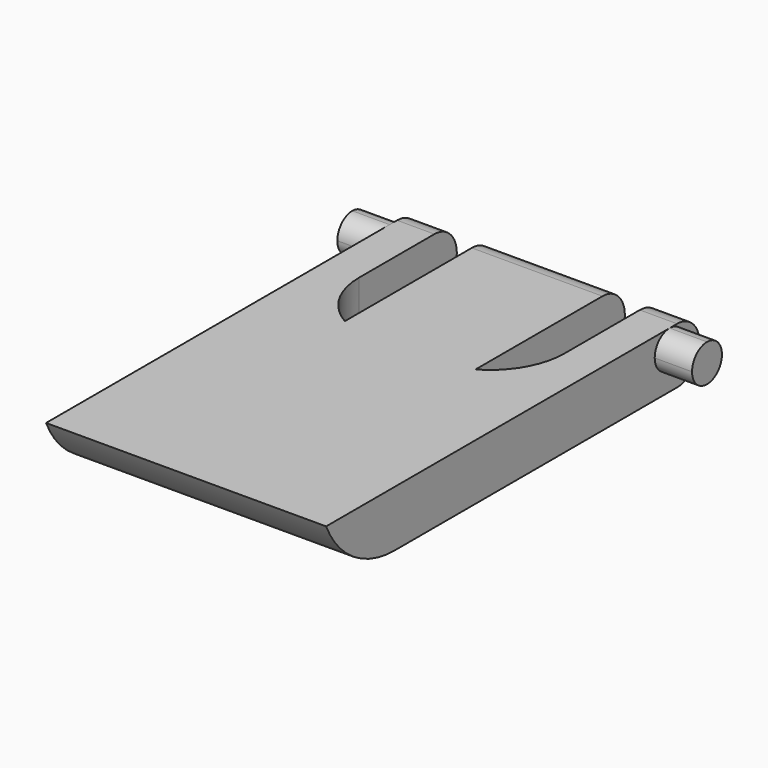
from build123d import *

# Parameters (mm, degrees)
F1_DEPTH    = 3
F3_DEPTH    = 2
F4_R        = 1.49999
F5_T1_DEPTH = 3
F6_T1_DEPTH = 30.4128784748


# Not quite as in the source:
# - a fillet or chamfer that OpenCascade refuses, or shapes differently, is made with other operations: its cross-section is extruded or revolved along the edge and cut away or added
# - a fillet or chamfer is up to 0.001 mm smaller than in the source, because OpenCascade refuses the exact size
# - a feature names something its author has since deleted; it is built from what else it names


with BuildPart() as f1:
    # F0 (on Top) → F1 (new body)
    with BuildSketch(Plane.XY):
        Polygon((-7.5, 12.5), (-7.5, -12.5), (0, -12.5), (0, 12.5), (-3.5, 12.5), (-3.5, 2.5), (-5.5, 2.5), (-5.5, 12.5), align=None)
    extrude(amount=F1_DEPTH)

    # F2 (on face) → F3 (join)
    with BuildSketch(Plane(origin=(-7.5, 0, 0), x_dir=(0, -1, 0), z_dir=(-1, 0, 0))):
        with BuildLine():
            ThreePointArc((-10.4999999883, 3), (-11.2071067853, 1.2928932229), (-9.5, 2))
            ThreePointArc((-9.5, 2), (-9.7928932147, 2.7071067771), (-10.4999999883, 3))
        make_face()
    extrude(amount=F3_DEPTH)

    # F4 (radius 1.5 in the source; OpenCascade refuses exactly that, so slightly less here)
    f4_edges = [f1.edges().sort_by_distance(p)[0] for p in [
        (-6.5, 12.5, 0),
        (-6.5, 12.5, 3),
        (-1.75, 12.5, 0),
        (-1.75, 12.5, 3),
    ]]
    fillet(f4_edges, radius=F4_R)

    # F5: fillet of radius 4 on 1 edges, made by hand

    # F5_s2 → F5_t1 (join)
    with BuildSketch(Plane.XY):
        with BuildLine():
            ThreePointArc((-5.5, 5.9641016151), (-4.9641016151, 3.9641016151), (-3.5, 2.5))
            Line((-3.5, 2.5), (-5.5, 2.5))
            Line((-5.5, 2.5), (-5.5, 5.9641016151))
        make_face()
    extrude(amount=F5_T1_DEPTH)

    # F6: fillet of radius 5 on 1 edges, made by hand

    # F6_s2 → F6_t1 (cut)
    with BuildSketch(Plane.YZ.offset(-18.9564392374)):
        with BuildLine():
            ThreePointArc((-7.917424305, 0), (-10.6560370926, 0.8166998673), (-12.5, 3))
            Line((-12.5, 3), (-12.5, 0))
            Line((-12.5, 0), (-7.917424305, 0))
        make_face()
    extrude(amount=F6_T1_DEPTH, mode=Mode.SUBTRACT)

    # F7: F1 across face


with BuildPart() as f1_1:
    add(f1.part)
    add(f1.part.mirror(Plane(origin=(0, 0.4580070694, 1.5370600849), x_dir=(0, 1, 0), z_dir=(1, 0, 0))))


solid = f1_1.part
